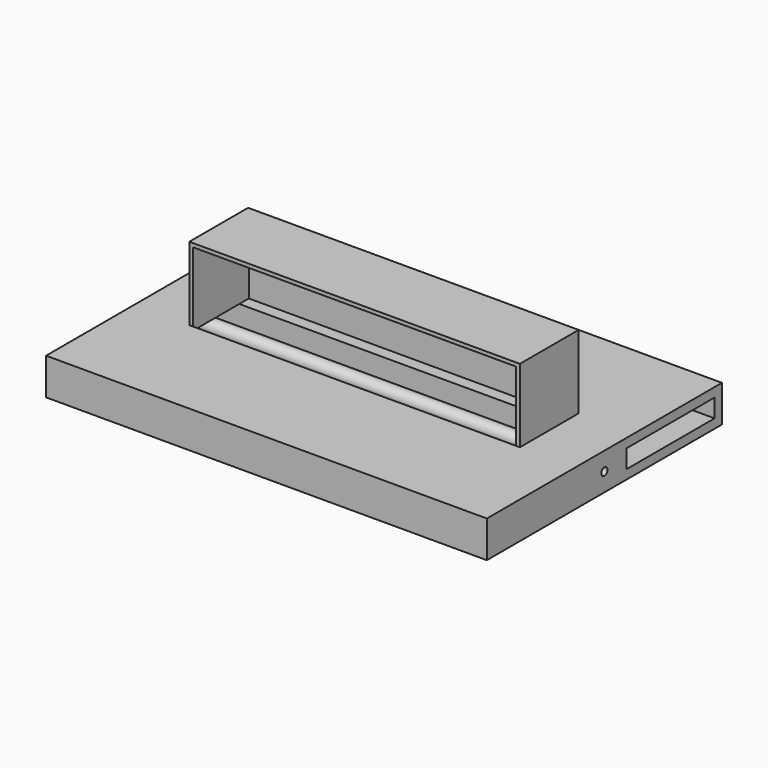
from build123d import *

# Parameters (mm, degrees)
F0_W           = 304.8
F0_H           = 203.2
F1_DEPTH       = 25.4
F2_W           = 76.2
F2_H           = 12.7
F3_DEPTH       = 378.206
F6_D           = 5.25
F6_CSINK_D     = 11.2
F6_CSINK_ANGLE = 90
F7_W           = 228.6
F7_H           = 50.8
F8_DEPTH       = 50.8
F9_T           = -2.54
F4_R           = 25.4
F13_DEPTH      = 25.4


# Not quite as in the source:
# - a shell that OpenCascade refuses in one call is made with other operations: the cavity is built on its own and cut out
# - the program builds the solid bodies; features that only make, move or delete a surface that nothing else refers to are left out


with BuildPart() as f1:
    # F0 (on Top) → F1 (new body)
    with BuildSketch(Plane.XY):
        Rectangle(F0_W, F0_H)
    extrude(amount=F1_DEPTH)

    # F2 (on face) → F3 (cut)
    with BuildSketch(Plane(origin=(-152.4, 0, 0), x_dir=(0, -1, 0), z_dir=(-1, 0, 0))):
        with Locations((-57.15, 12.7)):
            Rectangle(F2_W, F2_H)
    extrude(amount=-F3_DEPTH, mode=Mode.SUBTRACT)

    # F6 (through all)
    with Locations(Plane(origin=(-152.4, 0, 0), x_dir=(0, -1, 0), z_dir=(-1, 0, 0))):
        with Locations((0, 12.7)):
            CounterSinkHole(F6_D / 2, F6_CSINK_D / 2, counter_sink_angle=F6_CSINK_ANGLE)

    # F7 (on face) → F8 (join)
    with BuildSketch(Plane.XY.offset(25.4)):
        Rectangle(F7_W, F7_H)
    extrude(amount=F8_DEPTH)

    # F9: a shell. OpenCascade refuses it in one call, so the cavity is built on its own and cut out:
    # the body offset inwards by the wall thickness, plus a prism from it out through each open face.
    f9_core = offset(f1.part, amount=F9_T, kind=Kind.INTERSECTION, mode=Mode.PRIVATE)
    f9_exits = [f9_core.faces().sort_by_distance(p)[0] for p in [
        (0, -22.86, 48.26),
    ]]
    add(f9_core, mode=Mode.SUBTRACT)
    extrude(f9_exits, amount=-F9_T, mode=Mode.SUBTRACT)

    # F4 (on face) → F13 (cut)
    with BuildSketch(Plane.XY.offset(25.4)):
        with Locations((-88.3831381798, 51.9134663045)):
            Circle(F4_R)
    extrude(amount=-F13_DEPTH, mode=Mode.SUBTRACT)


solid = f1.part
